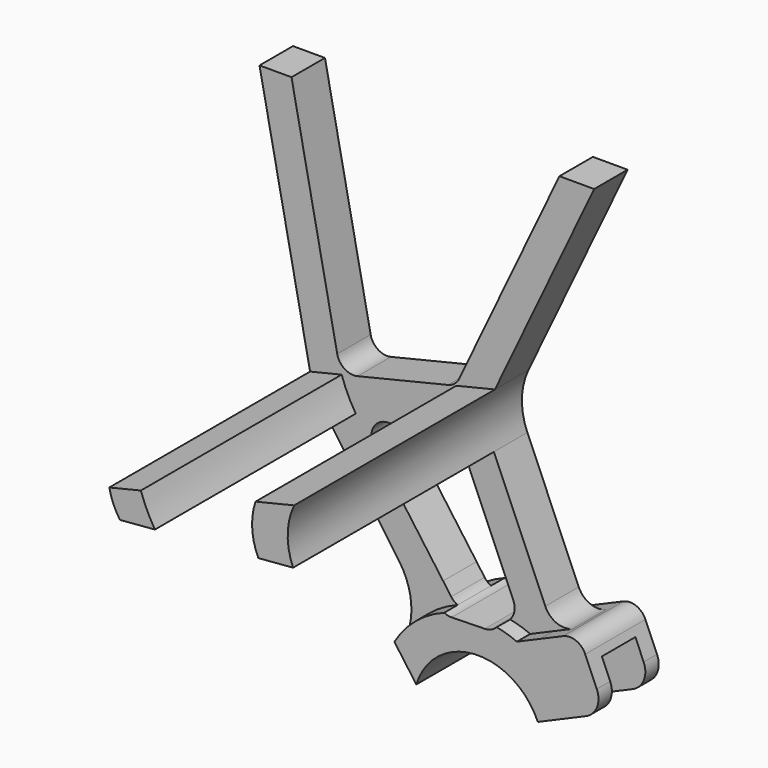
from build123d import *

# Parameters (mm, degrees)
F1_DEPTH      = 10
F3_DEPTH      = 4
F3_DEPTH_BACK = 14
F4_W          = 10
F4_H          = 10
F5_DEPTH      = 25
F6_T1_DEPTH   = 10
F7_R          = 4
F8_R          = 5
F10_DEPTH     = 60


# Not quite as in the source:
# - a fillet or chamfer that OpenCascade refuses, or shapes differently, is made with other operations: its cross-section is extruded or revolved along the edge and cut away or added
# - a feature names something its author has since deleted; it is built from what else it names


with BuildPart() as f1:
    # F0 (on Front) → F1 (new body)
    with BuildSketch(Plane.XZ):
        with BuildLine():
            ThreePointArc((19.6522871604, -43.3779198274), (22.0356929141, -43.9481357221), (24.344898549, -44.7687077723))
            Line((24.344898549, -44.7687077723), (30.2937477303, -42.2061976958))
            Line((30.2937477303, -42.2061976958), (16.0343749186, -9.1031636608))
            ThreePointArc((16.0343749186, -9.1031636608), (14.7317766807, -2.4774455359), (16.2784975378, 4.0955718405))
            Line((16.2784975378, 4.0955718405), (40, 54))
            Line((40, 54), (31.6958138155, 54))
            Line((31.6958138155, 54), (7.7256415471, 3.5724294089))
            ThreePointArc((7.7256415471, 3.5724294089), (6.6322171557, 2.1826346144), (5.0464276278, 1.4000887411))
            Line((5.0464276278, 1.4000887411), (-16.5758134292, -3.788837771))
            ThreePointArc((-16.5758134292, -3.788837771), (-19.6646678264, -3.268857876), (-21.4317839616, -0.6826055404))
            Line((-21.4317839616, -0.6826055404), (-32.3519113749, 54))
            Line((-32.3519113749, 54), (-40, 54))
            Line((-40, 54), (-27.9160834498, -6.5102868387))
            ThreePointArc((-27.9160834498, -6.5102868387), (-26.9490490541, -9.6402216111), (-25.3648124606, -12.5075969995))
            Line((-25.3648124606, -12.5075969995), (-6.5550611463, -39.5746751924))
            ThreePointArc((-6.5550611463, -39.5746751924), (-4.9098360692, -42.5874005907), (-3.945102256, -45.8817242769))
            Line((-3.945102256, -45.8817242769), (3.8871387568, -40.2303608977))
            Line((3.8871387568, -40.2303608977), (-12.4880276922, -17.5359698901))
            ThreePointArc((-12.4880276922, -17.5359698901), (-12.8770477363, -13.5212266501), (-9.5721086698, -11.2088950032))
            Line((-9.5721086698, -11.2088950032), (5.2830699548, -9.987289736))
            ThreePointArc((5.2830699548, -9.987289736), (7.6708908871, -10.5450664651), (9.284566981, -12.3913744428))
            Line((9.284566981, -12.3913744428), (20.6643672802, -38.8095010734))
            ThreePointArc((20.6643672802, -38.8095010734), (20.8960138101, -41.2571363473), (19.6522871604, -43.3779198274))
        make_face()
        with BuildLine():
            Line((-4.3718418374, -54.4194170272), (-2.8750095458, -56.4938812719))
            Line((-2.8750095458, -56.4938812719), (24.344898549, -44.7687077723))
            ThreePointArc((24.344898549, -44.7687077723), (22.0356929141, -43.9481357221), (19.6522871604, -43.3779198274))
            ThreePointArc((19.6522871604, -43.3779198274), (18.4554525804, -44.1141232898), (17.0778668556, -44.3910097661))
            Line((17.0778668556, -44.3910097661), (9.1481831441, -44.5638505003))
            ThreePointArc((9.1481831441, -44.5638505003), (8.440161238, -44.5163238476), (7.7516789791, -44.3444344023))
            ThreePointArc((7.7516789791, -44.3444344023), (0.7998412321, -48.3108696597), (-4.3718418374, -54.4194170272))
        make_face()
        with BuildLine():
            Line((-4.5614236042, -54.156675103), (-4.3718418374, -54.4194170272))
            ThreePointArc((-4.3718418374, -54.4194170272), (0.7998412321, -48.3108696597), (7.7516789791, -44.3444344023))
            ThreePointArc((7.7516789791, -44.3444344023), (6.6734648322, -43.7740983951), (5.81726752, -42.9053319878))
            Line((5.81726752, -42.9053319878), (3.8871387568, -40.2303608977))
            Line((3.8871387568, -40.2303608977), (-3.945102256, -45.8817242769))
            ThreePointArc((-3.945102256, -45.8817242769), (-3.7026448472, -49.2316692283), (-4.1648631271, -52.5584200507))
            Line((-4.1648631271, -52.5584200507), (-4.5614236042, -54.156675103))
        make_face()
        Polygon((30.2937477303, -42.2061976958), (36.6235819074, -56.9008633705), (45.807747954, -52.9447170098), (39.477913777, -38.2500513351), align=None)
        with BuildLine():
            ThreePointArc((24.344898549, -44.7687077723), (31.6655422142, -49.6392162498), (36.6235819074, -56.9008633705))
            Line((36.6235819074, -56.9008633705), (30.2937477303, -42.2061976958))
            Line((30.2937477303, -42.2061976958), (24.344898549, -44.7687077723))
        make_face()
    extrude(amount=F1_DEPTH)

    # F2 (on face) → F3 (join, two sides)
    with BuildSketch(Plane.XZ.offset(10)) as f3_sk:
        with BuildLine():
            Line((45.807747954, -52.9447170098), (39.477913777, -38.2500513351))
            Line((39.477913777, -38.2500513351), (30.2937477303, -42.2061976958))
            Line((30.2937477303, -42.2061976958), (24.721675481, -44.6064083669))
            ThreePointArc((24.721675481, -44.6064083669), (31.9751079214, -49.5289380846), (36.8958559524, -56.7835793441))
            Line((36.8958559524, -56.7835793441), (45.807747954, -52.9447170098))
        make_face()
        with BuildLine():
            Line((36.6235819074, -56.9008633705), (36.8958559524, -56.7835793441))
            ThreePointArc((36.8958559524, -56.7835793441), (31.9751079214, -49.5289380846), (24.721675481, -44.6064083669))
            ThreePointArc((24.721675481, -44.6064083669), (22.3566538827, -43.7354236695), (19.9113834301, -43.1250189536))
            ThreePointArc((19.9113834301, -43.1250189536), (18.6224089936, -44.0440177459), (17.0778668556, -44.3910097661))
            Line((17.0778668556, -44.3910097661), (9.1481831441, -44.5638505003))
            ThreePointArc((9.1481831441, -44.5638505003), (8.2237355637, -44.4761887941), (7.3444115948, -44.177730654))
            ThreePointArc((7.3444115948, -44.177730654), (0.5352155123, -48.1455807465), (-4.5614236042, -54.156675103))
            Line((-4.5614236042, -54.156675103), (-2.8750095458, -56.4938812719))
            Line((-2.8750095458, -56.4938812719), (24.344898549, -44.7687077723))
            ThreePointArc((24.344898549, -44.7687077723), (31.6655422142, -49.6392162498), (36.6235819074, -56.9008633705))
        make_face()
        with BuildLine():
            Line((29.7354573724, -59.867973141), (36.6235819074, -56.9008633705))
            ThreePointArc((36.6235819074, -56.9008633705), (31.6655422142, -49.6392162498), (24.344898549, -44.7687077723))
            Line((24.344898549, -44.7687077723), (-2.8750095458, -56.4938812719))
            Line((-2.8750095458, -56.4938812719), (0.6883118522, -61.4322988045))
            ThreePointArc((0.6883118522, -61.4322988045), (14.6664598558, -50.5224287814), (29.7354573724, -59.867973141))
        make_face()
    extrude(amount=F3_DEPTH)
    extrude(f3_sk.sketch, amount=-F3_DEPTH_BACK)

    # F4 (on face) → F5 (cut)
    with BuildSketch(Plane(origin=(19.4014510262, 0, 8.35731622), x_dir=(0, 1, 0), z_dir=(0.9184166047, 0, 0.3956146361))):
        with Locations((-5, -61.7475227671)):
            Rectangle(F4_W, F4_H)
    extrude(amount=-F5_DEPTH, mode=Mode.SUBTRACT)

    # F6: fillet of radius 5 on 1 edges, made by hand

    # F6_s2 → F6_t1 (join)
    with BuildSketch(Plane.XZ):
        with BuildLine():
            ThreePointArc((28.31567455, -37.6141146724), (31.0593734872, -40.2818434972), (34.8858307536, -40.2281245155))
            Line((34.8858307536, -40.2281245155), (30.2937477303, -42.2061976958))
            Line((30.2937477303, -42.2061976958), (28.31567455, -37.6141146724))
        make_face()
    extrude(amount=F6_T1_DEPTH)

    # F7
    f7_edges = [f1.edges().sort_by_distance(p)[0] for p in [
        (39.477914, -5, -38.250051),
    ]]
    fillet(f7_edges, radius=F7_R)

    # F8
    f8_edges = [f1.edges().sort_by_distance(p)[0] for p in [
        (45.807748, -12, -52.944717),
        (45.807748, 2, -52.944717),
    ]]
    fillet(f8_edges, radius=F8_R)

    # F9 (on face) → F10 (join)
    with BuildSketch(Plane.XZ.offset(10)):
        with BuildLine():
            ThreePointArc((-17.0067008, -11.8202735087), (-18.8974369177, -8.3589640964), (-20.3653347512, -4.6982507964))
            Line((-20.3653347512, -4.6982507964), (-27.9160834498, -6.5102868387))
            ThreePointArc((-27.9160834498, -6.5102868387), (-26.9490490541, -9.6402216111), (-25.3648124606, -12.5075969995))
            Line((-25.3648124606, -12.5075969995), (-17.0067008, -11.8202735087))
        make_face()
        with BuildLine():
            Line((16.2784975378, 4.0955718405), (7.0391568902, 1.8783058544))
            ThreePointArc((7.0391568902, 1.8783058544), (6.2442508473, -4.0206259595), (7.72081337, -9.7868236042))
            Line((7.72081337, -9.7868236042), (16.0343749186, -9.1031636608))
            ThreePointArc((16.0343749186, -9.1031636608), (14.7317766807, -2.4774455359), (16.2784975378, 4.0955718405))
        make_face()
    extrude(amount=F10_DEPTH)


solid = f1.part
